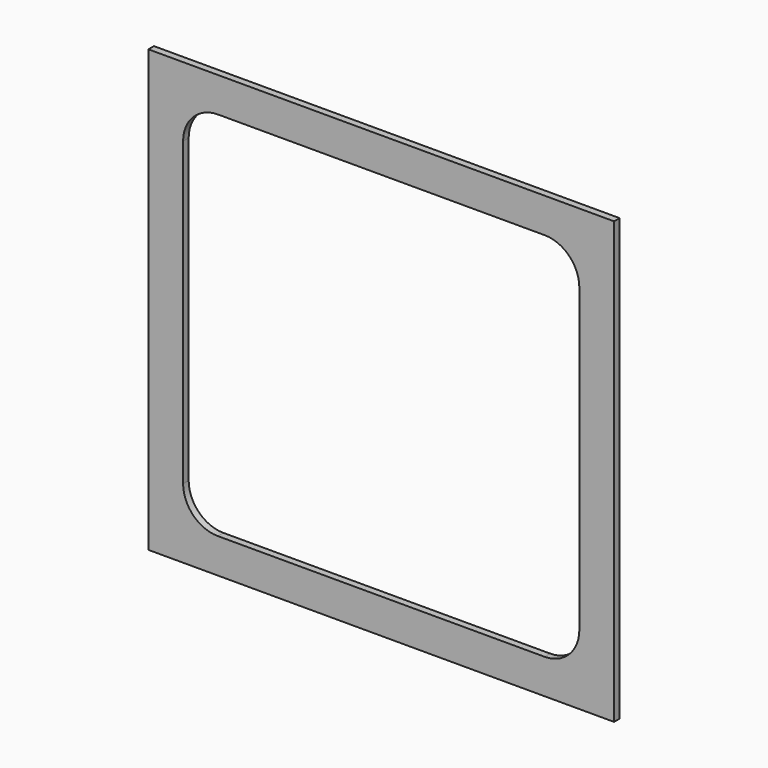
from build123d import *

# Parameters (mm, degrees)
F0_W     = 670
F0_H     = 634
F1_DEPTH = 10


# Not quite as in the source:
# - a feature names something its author has since deleted; it is built from what else it names


with BuildPart() as f1:
    # F0 (on Front) → F1 (new body)
    with BuildSketch(Plane.XZ):
        with Locations((-6.3475316763, 87.0849853243)):
            Rectangle(F0_W, F0_H)
        with BuildLine():
            ThreePointArc((-291.3475316763, 304.0849853243), (-276.7028707356, 339.4403243836), (-241.3475316763, 354.0849853243))
            Line((-241.3475316763, 354.0849853243), (228.6524683237, 354.0849853243))
            ThreePointArc((228.6524683237, 354.0849853243), (264.007807383, 339.4403243836), (278.6524683237, 304.0849853243))
            Line((278.6524683237, 304.0849853243), (278.6524683237, -129.9150146759))
            ThreePointArc((278.6524683237, -129.9150146759), (264.007807383, -165.2703537352), (228.6524683237, -179.9150146759))
            Line((228.6524683237, -179.9150146759), (-241.3475316763, -179.9150146759))
            ThreePointArc((-241.3475316763, -179.9150146759), (-276.7028707356, -165.2703537352), (-291.3475316763, -129.9150146759))
            Line((-291.3475316763, -129.9150146759), (-291.3475316763, 304.0849853243))
        make_face(mode=Mode.SUBTRACT)
    extrude(amount=F1_DEPTH)


solid = f1.part
